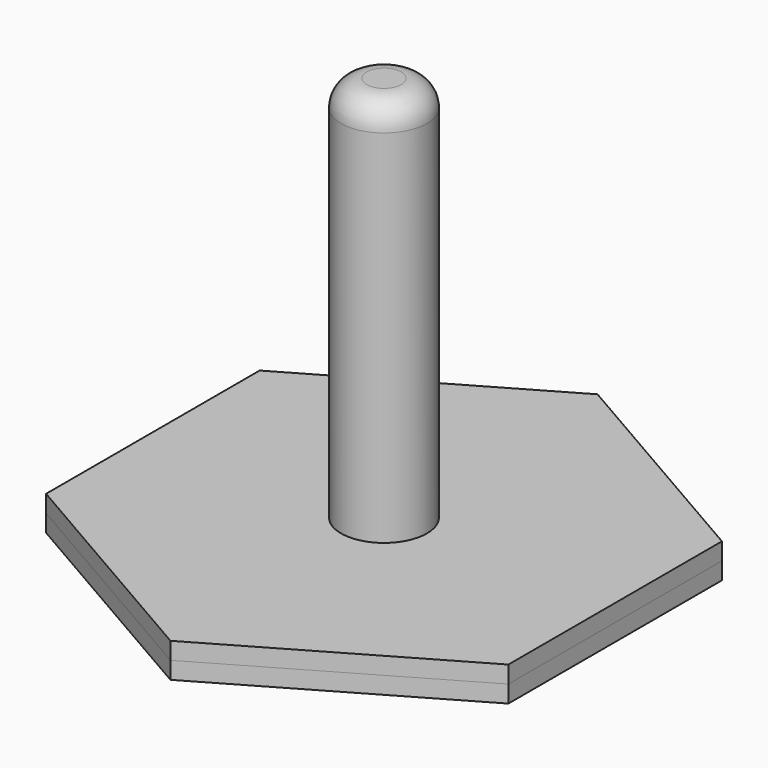
from build123d import *

# Parameters (mm, degrees)
F0_R     = 22.4
F1_DEPTH = 2
F2_R     = 5
F3_DEPTH = 45
F4_R     = 3
F5_DEPTH = 2
F6_DEPTH = 2


# Not quite as in the source:
# - a feature names something its author has since deleted; it is built from what else it names


with BuildPart() as f1:
    # F0 (on Top) → F1 (new body)
    with BuildSketch(Plane.XY):
        Polygon((26.9, -15.5307222412), (26.9, 15.5307222412), (0, 31.0614444824), (-26.9, 15.5307222412), (-26.9, -15.5307222412), (0, -31.0614444824), align=None)
        Circle(F0_R, mode=Mode.SUBTRACT)
        Circle(F0_R)
    extrude(amount=F1_DEPTH)

    # F2 (on face) → F3 (join)
    with BuildSketch(Plane.XY.offset(2)):
        Circle(F2_R)
    extrude(amount=F3_DEPTH)

    # F4
    f4_edges = [f1.edges().sort_by_distance(p)[0] for p in [
        (-5, 0, 47),
    ]]
    fillet(f4_edges, radius=F4_R)

    # F0 (on Top) → F5 (join)
    with BuildSketch(Plane.XY):
        Circle(F0_R)
    extrude(amount=-F5_DEPTH)


with BuildPart() as f6:
    # F0 (on Top) → F6 (new body)
    with BuildSketch(Plane.XY):
        Polygon((26.9, -15.5307222412), (26.9, 15.5307222412), (0, 31.0614444824), (-26.9, 15.5307222412), (-26.9, -15.5307222412), (0, -31.0614444824), align=None)
        Circle(F0_R, mode=Mode.SUBTRACT)
    extrude(amount=-F6_DEPTH)


solid = Compound([f1.part, f6.part])
